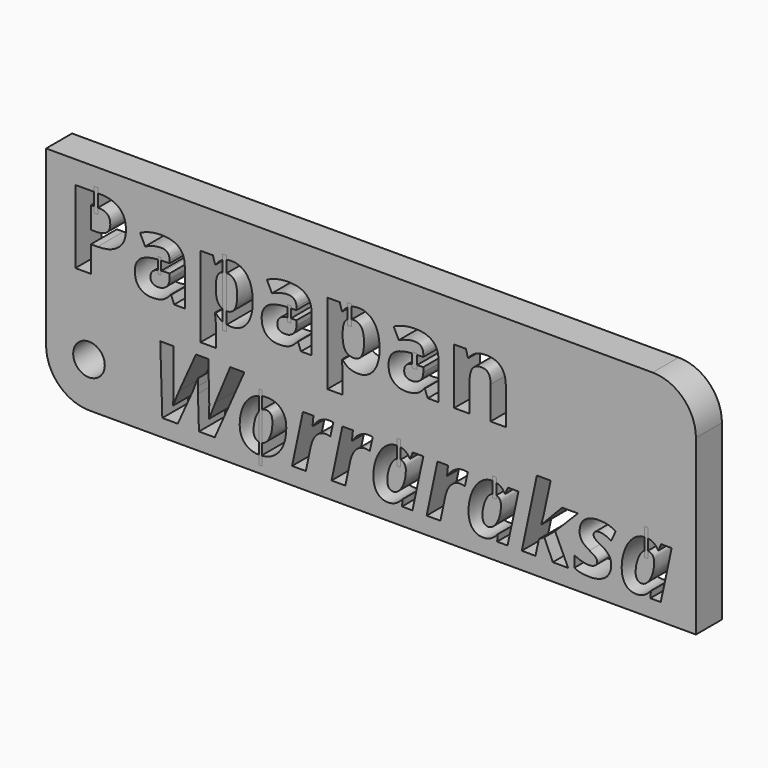
from build123d import *

# Parameters (mm, degrees)
F0_W           = 76.2
F0_H           = 25.4
F1_DEPTH       = 3.81
F2_TEXT_SIZE   = 12.0237702504
F2_TEXT_SIZE_2 = 10.9858924083
F3_DEPTH       = 3.811
F4_W           = 0.3815991804
F4_H           = 1.8199328333
F5_DEPTH       = 3.81
F4_W_2         = 0.499015674
F4_H_2         = 7.8961653635
F4_W_3         = 0.3816001117
F4_H_3         = 1.7905794084
F4_W_4         = 0.4403069615
F4_H_4         = 2.3483019322
F4_W_5         = 0.5577243865
F4_H_5         = 1.6731657088
F4_W_6         = 0.3522448242
F4_H_6         = 7.8668107162
F4_W_7         = 0.410951674
F4_H_7         = 2.8473157436
F4_H_8         = 2.2602402605
F4_H_9         = 3.1995610334
F4_W_8         = 0.4403064959
F4_H_10        = 2.7592554688
F6_R           = 1.8508000108
F7_DEPTH       = 3.8110001
F8_R           = 5.08
F9_R           = 5.08


# Not quite as in the source:
# - Text() gives the source's letters only with a copy of the font that has no kerning and outlines rounded to 1/6400 em; it was checked with that copy


with BuildPart() as f1:
    # F0 (on Front) → F1 (new body)
    with BuildSketch(Plane.XZ):
        with Locations((38.1, 12.7)):
            Rectangle(F0_W, F0_H)
    extrude(amount=F1_DEPTH)

    # F2 (on face) → F3 (cut, through all)
    with BuildSketch(Plane.XZ.offset(3.81)):
        with Locations((2.3544919677, 14.1661250964)):
            Text('Papapan', F2_TEXT_SIZE, font='Open Sans', font_style=FontStyle.BOLD, text_align=(TextAlign.LEFT, TextAlign.BOTTOM))
        with Locations((12.3996557668, 2.0081561524)):
            Text('Worraraksa', F2_TEXT_SIZE_2, font='Open Sans', font_style=FontStyle.BOLDITALIC, text_align=(TextAlign.LEFT, TextAlign.BOTTOM))
    extrude(amount=-F3_DEPTH, mode=Mode.SUBTRACT)

    # F6 (on face) → F7 (cut, through all)
    with BuildSketch(Plane.XZ.offset(3.81)):
        with Locations((5.0320662558, 5.2533536218)):
            Circle(F6_R)
    extrude(amount=-F7_DEPTH, mode=Mode.SUBTRACT)

    # F8
    f8_edges = [f1.edges().sort_by_distance(p)[0] for p in [
        (0, -1.905, 0),
    ]]
    fillet(f8_edges, radius=F8_R)

    # F9
    f9_edges = [f1.edges().sort_by_distance(p)[0] for p in [
        (76.2, -1.905, 25.4),
    ]]
    fillet(f9_edges, radius=F9_R)


with BuildPart() as f5:
    # F4 (on Front) → F5 (new body)
    with BuildSketch(Plane.XZ):
        with Locations((13.3025958203, 17.6111506298)):
            Rectangle(F4_W, F4_H)
    extrude(amount=F5_DEPTH)


with BuildPart() as f5b:
    # F4 (on Front) → F5, piece 2 (new body)
    with BuildSketch(Plane.XZ):
        with Locations((20.9345771, 17.3029364087)):
            Rectangle(F4_W_2, F4_H_2)
    extrude(amount=F5_DEPTH)


with BuildPart() as f5c:
    # F4 (on Front) → F5, piece 3 (new body)
    with BuildSketch(Plane.XZ):
        with Locations((28.5078510642, 17.5964739174)):
            Rectangle(F4_W_3, F4_H_3)
    extrude(amount=F5_DEPTH)


with BuildPart() as f5d:
    # F4 (on Front) → F5, piece 4 (new body)
    with BuildSketch(Plane.XZ):
        with Locations((35.5821102858, 19.8126835749)):
            Rectangle(F4_W_4, F4_H_4)
    extrude(amount=F5_DEPTH)


with BuildPart() as f5e:
    # F4 (on Front) → F5, piece 5 (new body)
    with BuildSketch(Plane.XZ):
        with Locations((43.2140920311, 17.5377670676)):
            Rectangle(F4_W_5, F4_H_5)
    extrude(amount=F5_DEPTH)


with BuildPart() as f5f:
    # F4 (on Front) → F5, piece 6 (new body)
    with BuildSketch(Plane.XZ):
        with Locations((25.1202080399, 4.7737594286)):
            Rectangle(F4_W_6, F4_H_6)
    extrude(amount=F5_DEPTH)


with BuildPart() as f5g:
    # F4 (on Front) → F5, piece 7 (new body)
    with BuildSketch(Plane.XZ):
        with Locations((41.3528457284, 7.4302759022)):
            Rectangle(F4_W_7, F4_H_7)
    extrude(amount=F5_DEPTH)


with BuildPart() as f5h:
    # F4 (on Front) → F5, piece 8 (new body)
    with BuildSketch(Plane.XZ):
        with Locations((52.580665797, 7.4889834505)):
            Rectangle(F4_W_4, F4_H_8)
    extrude(amount=F5_DEPTH)


with BuildPart() as f5i:
    # F4 (on Front) → F5, piece 9 (new body)
    with BuildSketch(Plane.XZ):
        with Locations((70.3543759882, 7.6063990127)):
            Rectangle(F4_W_7, F4_H_9)
    extrude(amount=F5_DEPTH)


with BuildPart() as f5j:
    # F4 (on Front) → F5, piece 10 (new body)
    with BuildSketch(Plane.XZ):
        with Locations((5.8621086646, 21.9447631389)):
            Rectangle(F4_W_8, F4_H_10)
    extrude(amount=F5_DEPTH)


solid = Compound([f1.part, f5.part, f5b.part, f5c.part, f5d.part, f5e.part, f5f.part, f5g.part, f5h.part, f5i.part, f5j.part])
